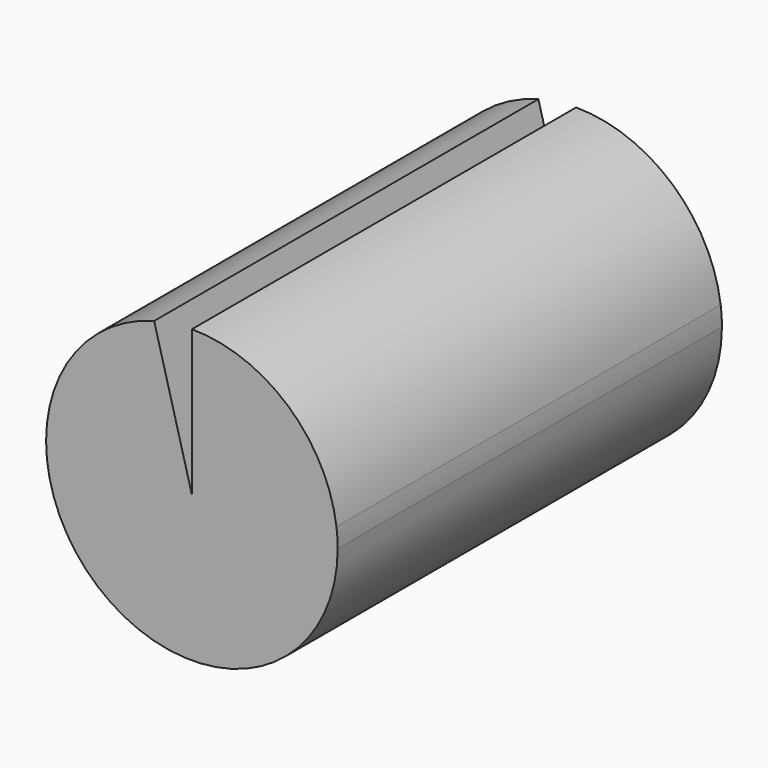
from build123d import *

# Parameters (mm, degrees)
F1_DEPTH = 56
F3_DEPTH = 56


# Not quite as in the source:
# - a feature of the source that left no trace in its solid (it failed there, or was rolled back) is left out
# - a feature names something its author has since deleted; it is built from what else it names


with BuildPart() as f1:
    # F0 (on Front) → F1 (new body)
    with BuildSketch(Plane.XZ):
        with BuildLine():
            ThreePointArc((17.0012298637, -0.0012299217), (17.0012298971, -0.0006149604), (17.0012299082, 8e-10))
            ThreePointArc((17.0012299082, 8e-10), (16.9647599435, 1.1129459753), (16.8555065268, 2.2211167615))
            Line((16.8555065268, 2.2211167615), (0.0018881159, 0.0022958043))
            Line((0.0018881159, 0.0022958043), (0.0009440615, 0.0021715172))
            Line((0.0009440615, 0.0021715172), (0.0012299082, 8e-10))
            Line((0.0012299082, 8e-10), (6.4e-09, 8e-10))
            Line((-3.33e-08, 8e-10), (-5.49e-08, -0.0012299217))
            Line((-5.49e-08, -0.0012299217), (17.0012298637, -0.0012299217))
        make_face()
        with BuildLine():
            Line((0.0018881159, 0.0022958043), (16.8555065268, 2.2211167615))
            ThreePointArc((16.8555065268, 2.2211167615), (11.2089354185, 12.7823056298), (0.0002990162, 16.9999999754))
            Line((0.0002990162, 16.9999999754), (1.31e-07, 0.0093423556))
            Line((1.31e-07, 0.0093423556), (0.0018881159, 0.0022958043))
        make_face()
        with BuildLine():
            ThreePointArc((-16.9987700918, 8e-10), (0.0006149469, -16.999999988), (17.0012298637, -0.0012299217))
            Line((17.0012298637, -0.0012299217), (-5.49e-08, -0.0012299217))
            Line((-5.49e-08, -0.0012299217), (-3.33e-08, 8e-10))
            Line((-3.33e-08, 8e-10), (2.7e-09, 0.0020472295))
            Line((2.7e-09, 0.0020472295), (1.31e-07, 0.0093423556))
            Line((1.31e-07, 0.0093423556), (-4.3972169489, 16.4211347133))
            ThreePointArc((-4.3972169489, 16.4211347133), (-13.4853114678, 10.3495507986), (-16.9987700918, 8e-10))
        make_face()
        Polygon((0.0009440615, 0.0021715172), (0.0018881159, 0.0022958043), (1.31e-07, 0.0093423556), align=None)
        Polygon((0.0009440615, 0.0021715172), (1.31e-07, 0.0093423556), (2.7e-09, 0.0020472295), align=None)
        Polygon((0.0012299082, 8e-10), (0.0009440615, 0.0021715172), (2.7e-09, 0.0020472295), (-3.33e-08, 8e-10), align=None)
    extrude(amount=F1_DEPTH)

    # F0 (on Front) → F3 (cut)
    with BuildSketch(Plane.XZ):
        with BuildLine():
            Line((1.31e-07, 0.0093423556), (0.0002990162, 16.9999999754))
            ThreePointArc((0.0002990162, 16.9999999754), (-1.1109385334, 16.9635810307), (-2.2174188682, 16.8546016754))
            Line((-2.2174188682, 16.8546016754), (1.31e-07, 0.0093423556))
        make_face()
        with BuildLine():
            Line((1.31e-07, 0.0093423556), (-2.2174188682, 16.8546016754))
            ThreePointArc((-2.2174188682, 16.8546016754), (-3.3144091037, 16.6735280601), (-4.3972169489, 16.4211347133))
            Line((-4.3972169489, 16.4211347133), (1.31e-07, 0.0093423556))
        make_face()
    extrude(amount=F3_DEPTH, mode=Mode.SUBTRACT)


solid = f1.part
